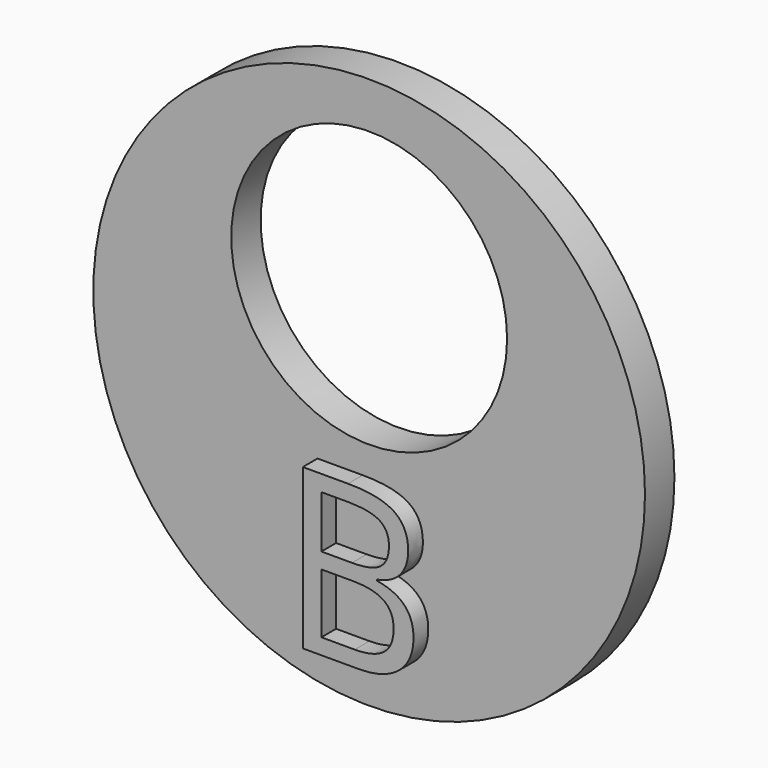
from build123d import *

# Parameters (mm, degrees)
F0_R         = 15
F0_R_2       = 7.5
F1_DEPTH     = 2
F2_TEXT_SIZE = 12.1644095985
F3_DEPTH     = 1


# Not quite as in the source:
# - Text() gives the source's letters only with a copy of the font that has no kerning and outlines rounded to 1/6400 em; it was checked with that copy


with BuildPart() as f1:
    # F0 (on Front) → F1 (new body)
    with BuildSketch(Plane.XZ):
        Circle(F0_R)
        with Locations((0, 5)):
            Circle(F0_R_2, mode=Mode.SUBTRACT)
    extrude(amount=F1_DEPTH)

    # F2 (on face) → F3 (join)
    with BuildSketch(Plane.XZ.offset(2)):
        with Locations((-4, -12.7583749109)):
            Text('B', F2_TEXT_SIZE, font='Open Sans', text_align=(TextAlign.LEFT, TextAlign.BOTTOM))
    extrude(amount=F3_DEPTH)


solid = f1.part
